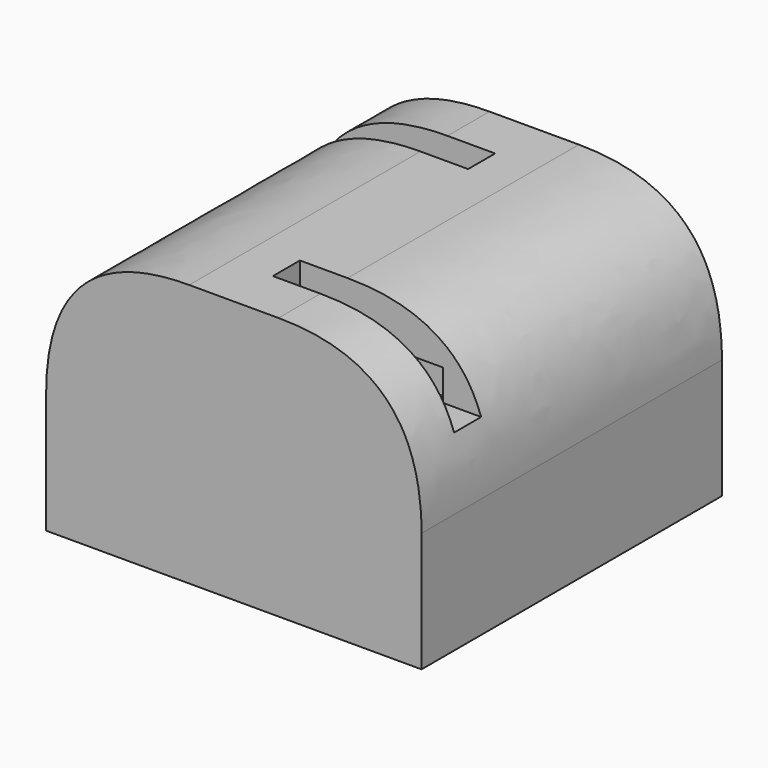
from build123d import *

# Parameters (mm, degrees)
F0_W        = 100
F0_H        = 70
F1_DEPTH    = 100
F2_T        = -12.7
F3_T1_DEPTH = 290.5
F4_T1_DEPTH = 290.5
F5_W        = 9
F5_H        = 32
F6_DEPTH    = 50.8
F7_W        = 9
F7_H        = 30
F8_DEPTH    = 50.8
F9_W        = 10
F9_H        = 10
F10_DEPTH   = 83.82


# Not quite as in the source:
# - a fillet or chamfer that OpenCascade refuses, or shapes differently, is made with other operations: its cross-section is extruded or revolved along the edge and cut away or added


with BuildPart() as f1:
    # F0 (on Front) → F1 (new body)
    with BuildSketch(Plane.XZ):
        with Locations((-15.9141167998, -52.9208671927)):
            Rectangle(F0_W, F0_H)
    extrude(amount=F1_DEPTH)

    # F2
    f2_openings = [f1.faces().sort_by_distance(p)[0] for p in [
        (-15.914117, -50, -87.920867),
    ]]
    offset(amount=F2_T, openings=f2_openings)

    # F3: fillet of radius 38.1 on 1 edges, made by hand

    # F3_s2 → F3_t1 (cut)
    with BuildSketch(Plane.XZ.offset(-95.25)):
        with BuildLine():
            add(Edge.make_bspline(
                [(34.0858832002, -56.0208671927), (34.0858832002, -17.9208671927), (-4.0141167998, -17.9208671927)],
                knots=[0, 0, 0, 1, 1, 1], degree=2, weights=[1, 1, 1]))
            Line((-4.0141167998, -17.9208671927), (34.0858832002, -17.9208671927))
            Line((34.0858832002, -17.9208671927), (34.0858832002, -56.0208671927))
        make_face()
    extrude(amount=F3_T1_DEPTH, mode=Mode.SUBTRACT)

    # F4: fillet of radius 38.1 on 1 edges, made by hand

    # F4_s2 → F4_t1 (cut)
    with BuildSketch(Plane.XZ.offset(-95.25)):
        with BuildLine():
            add(Edge.make_bspline(
                [(-27.8141167998, -17.9208671927), (-65.9141167998, -17.9208671927), (-65.9141167998, -56.0208671927)],
                knots=[0, 0, 0, 1, 1, 1], degree=2, weights=[1, 1, 1]))
            Line((-65.9141167998, -56.0208671927), (-65.9141167998, -17.9208671927))
            Line((-65.9141167998, -17.9208671927), (-27.8141167998, -17.9208671927))
        make_face()
    extrude(amount=F4_T1_DEPTH, mode=Mode.SUBTRACT)

    # F5 (on face) → F6 (cut)
    with BuildSketch(Plane(origin=(-65.9141167998, 0, 0), x_dir=(0, -1, 0), z_dir=(-1, 0, 0))):
        with Locations((18.5, -22.9208671927)):
            Rectangle(F5_W, F5_H)
    extrude(amount=-F6_DEPTH, mode=Mode.SUBTRACT)

    # F7 (on face) → F8 (cut)
    with BuildSketch(Plane.YZ.offset(34.0858832002)):
        with Locations((-81.5, -23.9208671927)):
            Rectangle(F7_W, F7_H)
    extrude(amount=-F8_DEPTH, mode=Mode.SUBTRACT)

    # F9 (on face) → F10 (join)
    with BuildSketch(Plane(origin=(21.3858832002, 0, 0), x_dir=(0, -1, 0), z_dir=(-1, 0, 0))):
        with Locations((25, -46.9208671927)):
            Rectangle(F9_W, F9_H)
        with Locations((75, -46.9208671927)):
            Rectangle(F9_W, F9_H)
    extrude(amount=F10_DEPTH)


solid = f1.part
